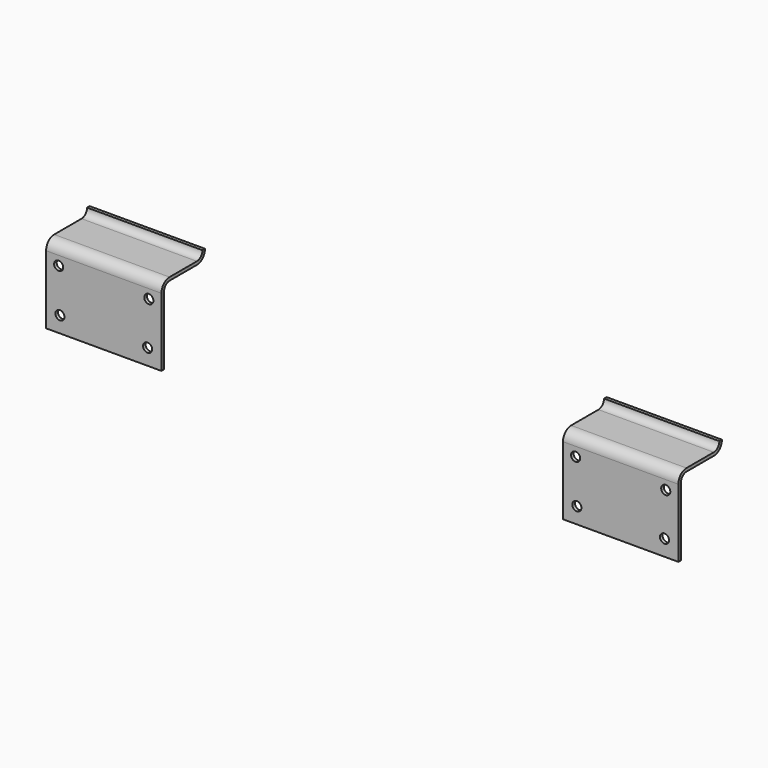
from build123d import *

# Parameters (mm, degrees)
F1_W = 171.45
F1_H = 4.7625
F6_D = 13.49248


with BuildPart() as f2:
    # F2: sweep along a path in F0
    with BuildLine(Plane.YZ) as f2_path:
        Line((0, 0), (0, 101.6))
        ThreePointArc((0, 101.6), (3.7197438789, 110.5802561211), (12.7, 114.3))
        Line((12.7, 114.3), (63.5, 114.3))
        ThreePointArc((63.5, 114.3), (72.4802561211, 118.0197438789), (76.2, 127))
    # F1 (on Top) → F2 (sweep)
    with BuildSketch(Plane.XY):
        Rectangle(F1_W, F1_H)
    sweep(path=f2_path.line)


with BuildPart() as f4_1:
    # F4: copy of F2
    add(f2.part.moved(Location((768.35, 0, 0))))


with BuildPart() as f2_1:
    add(f2.part)

    # F6 (through all)
    with Locations(Plane.XZ.offset(2.38125)):
        with Locations((-67.0052, 87.9475), (67.0052, 87.9475), (65.1383, 23.8125), (-65.1383, 23.8125)):
            Hole(F6_D / 2)


with BuildPart() as f7_1:
    # F7: copy of F2
    add(f2_1.part.moved(Location((384.175, 0, 0))))


with BuildPart() as f2_2:
    # F8: moved
    add(f2_1.part.moved(Location((-384.175, 0, 0))))


solid = Compound([f7_1.part, f2_2.part])
